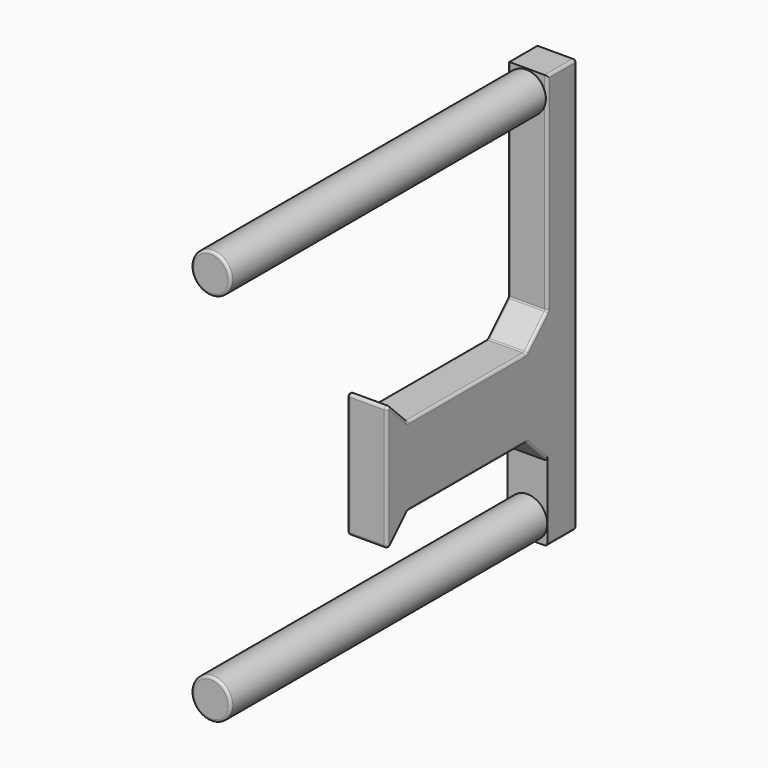
from build123d import *

# Parameters (mm, degrees)
F0_R     = 3.75
F1_DEPTH = 75
F2_W     = 7.5
F2_H     = 78.5
F3_DEPTH = 7
F4_W     = 7.5
F4_H     = 25
F5_DEPTH = 45
F7_DEPTH = 25
F8_R     = 0.5
F8_2_R   = 0.5
F8_3_R   = 0.5


with BuildPart() as f1:
    # F0 (on Front) → F1 (new body)
    with BuildSketch(Plane.XZ):
        with Locations((0, 35.5)):
            Circle(F0_R)
    extrude(amount=F1_DEPTH)

    # F8
    f8_edges = [f1.edges().sort_by_distance(p)[0] for p in [
        (-3.75, -75, 35.5),
        (3.75, -37.5, 35.5),
        (-3.75, 0, 35.5),
    ]]
    fillet(f8_edges, radius=F8_R)


with BuildPart() as f1b:
    # F0 (on Front) → F1, piece 2 (new body)
    with BuildSketch(Plane.XZ):
        with Locations((0, -35.5)):
            Circle(F0_R)
    extrude(amount=F1_DEPTH)

    # F8#2
    f8_2_edges = [f1b.edges().sort_by_distance(p)[0] for p in [
        (-3.75, -75, -35.5),
    ]]
    fillet(f8_2_edges, radius=F8_2_R)


with BuildPart() as f3:
    # F2 (on Front) → F3 (new body)
    with BuildSketch(Plane.XZ):
        Rectangle(F2_W, F2_H)
    extrude(amount=-F3_DEPTH)

    # F4 (on face) → F5 (join)
    with BuildSketch(Plane(origin=(0, 7, 0), x_dir=(-1, 0, 0), z_dir=(0, 1, 0))):
        with Locations((0, -12.5)):
            Rectangle(F4_W, F4_H)
    extrude(amount=-F5_DEPTH)

    # F6 (on face) → F7 (cut)
    with BuildSketch(Plane.YZ.offset(3.75)):
        Polygon((0, 0), (-38, 0), (-33, -5), (-5, -5), align=None)
        Polygon((-33, -20), (-38, -25), (0, -25), (-5, -20), align=None)
    extrude(amount=-F7_DEPTH, mode=Mode.SUBTRACT)

    # F8#3
    f8_3_edges = [f3.edges().sort_by_distance(p)[0] for p in [
        (-3.75, 3.5, -39.25),
        (0, 7, -39.25),
        (3.75, 3.5, -39.25),
        (-3.75, 7, 0),
        (3.75, 7, 0),
        (3.75, -19, -20),
        (3.75, -2.5, -22.5),
        (-3.75, -2.5, -22.5),
        (-3.75, -19, -20),
        (0, -5, -20),
        (0, 0, 0),
        (0, -5, -5),
        (3.75, -2.5, -2.5),
        (3.75, -19, -5),
        (-3.75, -2.5, -2.5),
        (-3.75, 0, 19.625),
        (-3.75, -35.5, -2.5),
        (0, 7, 39.25),
        (3.75, 3.5, 39.25),
        (-3.75, 3.5, 39.25),
        (0, -38, -25),
        (0, -38, 0),
        (3.75, -38, -12.5),
        (-3.75, -38, -12.5),
        (3.75, -35.5, -22.5),
        (-3.75, -35.5, -22.5),
        (0, -33, -20),
        (3.75, -35.5, -2.5),
        (0, -33, -5),
        (3.75, 0, 19.625),
        (-3.75, -19, -5),
    ]]
    fillet(f8_3_edges, radius=F8_3_R)


solid = Compound([f1.part, f1b.part, f3.part])
